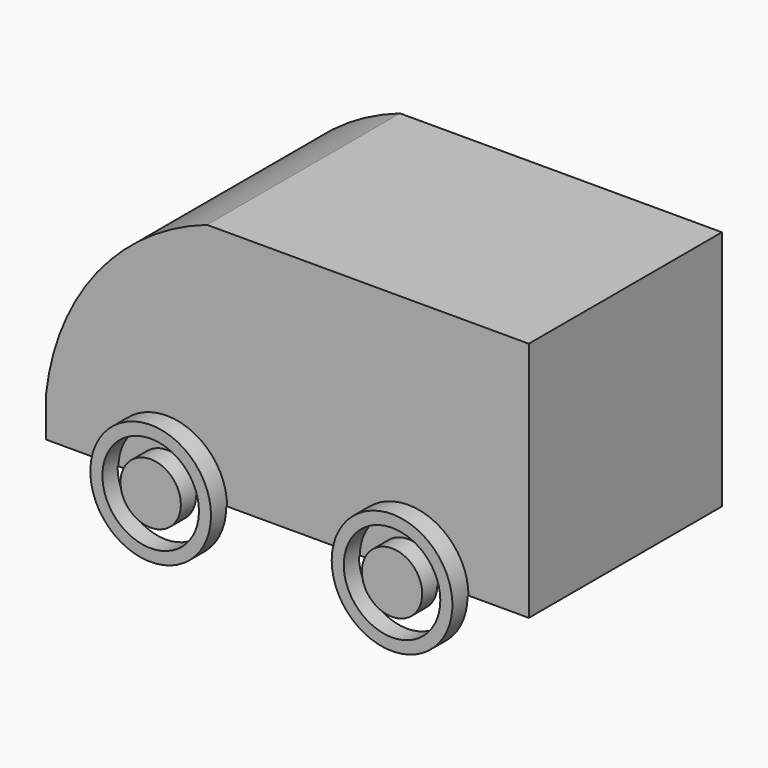
from build123d import *

# Parameters (mm, degrees)
F1_DEPTH = 76.2
F2_R     = 15.24
F3_DEPTH = 6.35
F2_R_2   = 9.525
F4_DEPTH = 6.35
F5_R     = 15.24
F6_DEPTH = 6.35
F5_R_2   = 9.525
F7_DEPTH = 6.35
F8_W     = 152.5372415781
F8_H     = 76.57238096
F9_DEPTH = 25.4


with BuildPart() as f1:
    # F0 (on Front) → F1 (new body)
    with BuildSketch(Plane.XZ):
        with BuildLine():
            Line((82.9111417405, 0), (101.9611417405, 0))
            Line((101.9611417405, 0), (101.9611417405, 76.2))
            Line((101.9611417405, 76.2), (0.3611417405, 76.2))
            ThreePointArc((0.3611417405, 76.2), (-34.2470067394, 51.816518784), (-50.4388582595, 12.7))
            Line((-50.4388582595, 12.7), (-50.4388582595, 0))
            Line((-50.4388582595, 0), (-31.3888582595, 0))
            ThreePointArc((-31.3888582595, 0), (-12.3388582595, 19.05), (6.7111417405, 0))
            Line((6.7111417405, 0), (44.8111417405, 0))
            ThreePointArc((44.8111417405, 0), (63.8611417405, 19.05), (82.9111417405, 0))
        make_face()
        with BuildLine():
            ThreePointArc((44.8111417405, 0), (63.8611417405, -19.05), (82.9111417405, 0))
            Line((82.9111417405, 0), (63.8611417405, 0))
            Line((63.8611417405, 0), (44.8111417405, 0))
        make_face()
        with BuildLine():
            Line((63.8611417405, 0), (82.9111417405, 0))
            ThreePointArc((82.9111417405, 0), (63.8611417405, 19.05), (44.8111417405, 0))
            Line((44.8111417405, 0), (63.8611417405, 0))
        make_face()
        with BuildLine():
            Line((-12.3388582595, 0), (6.7111417405, 0))
            ThreePointArc((6.7111417405, 0), (-12.3388582595, 19.05), (-31.3888582595, 0))
            Line((-31.3888582595, 0), (-12.3388582595, 0))
        make_face()
        with BuildLine():
            ThreePointArc((-31.3888582595, 0), (-12.3388582595, -19.05), (6.7111417405, 0))
            Line((6.7111417405, 0), (-12.3388582595, 0))
            Line((-12.3388582595, 0), (-31.3888582595, 0))
        make_face()
    extrude(amount=F1_DEPTH)

    # F2 (on face) → F3 (join)
    with BuildSketch(Plane.XZ.offset(76.2)):
        with BuildLine():
            ThreePointArc((82.9111417405, 0), (63.8611417405, 19.05), (44.8111417405, 0))
            ThreePointArc((44.8111417405, 0), (63.8611417405, -19.05), (82.9111417405, 0))
        make_face()
        with Locations((63.8611417405, 0)):
            Circle(F2_R, mode=Mode.SUBTRACT)
        with BuildLine():
            ThreePointArc((-31.3888582595, 0), (-12.3388582595, -19.05), (6.7111417405, 0))
            ThreePointArc((6.7111417405, 0), (-12.3388582595, 19.05), (-31.3888582595, 0))
        make_face()
        with Locations((-12.3388582595, 0)):
            Circle(F2_R, mode=Mode.SUBTRACT)
    extrude(amount=F3_DEPTH)

    # F2 (on face) → F4 (join)
    with BuildSketch(Plane.XZ.offset(76.2)):
        with Locations((63.8611417405, 0)):
            Circle(F2_R_2)
        with Locations((-12.3388582595, 0)):
            Circle(F2_R_2)
    extrude(amount=F4_DEPTH)

    # F5 (on face) → F6 (join)
    with BuildSketch(Plane(origin=(0, 0, 0), x_dir=(-1, 0, 0), z_dir=(0, 1, 0))):
        with BuildLine():
            ThreePointArc((-82.9111417405, 0), (-63.8611417405, -19.05), (-44.8111417405, 0))
            ThreePointArc((-44.8111417405, 0), (-63.8611417405, 19.05), (-82.9111417405, 0))
        make_face()
        with Locations((-63.8611417405, 0)):
            Circle(F5_R, mode=Mode.SUBTRACT)
        with BuildLine():
            ThreePointArc((31.3888582595, 0), (12.3388582595, 19.05), (-6.7111417405, 0))
            ThreePointArc((-6.7111417405, 0), (12.3388582595, -19.05), (31.3888582595, 0))
        make_face()
        with Locations((12.3388582595, 0)):
            Circle(F5_R, mode=Mode.SUBTRACT)
    extrude(amount=F6_DEPTH)

    # F5 (on face) → F7 (join)
    with BuildSketch(Plane(origin=(0, 0, 0), x_dir=(-1, 0, 0), z_dir=(0, 1, 0))):
        with Locations((-63.8611417405, 0)):
            Circle(F5_R_2)
        with Locations((12.3388582595, 0)):
            Circle(F5_R_2)
    extrude(amount=F7_DEPTH)

    # F8 (on face) → F9 (cut)
    with BuildSketch(Plane(origin=(0, 0, 0), x_dir=(1, 0, 0), z_dir=(0, 0, -1))):
        with Locations((25.47326684, 38.28619048)):
            Rectangle(F8_W, F8_H)
    extrude(amount=F9_DEPTH, mode=Mode.SUBTRACT)


solid = f1.part
